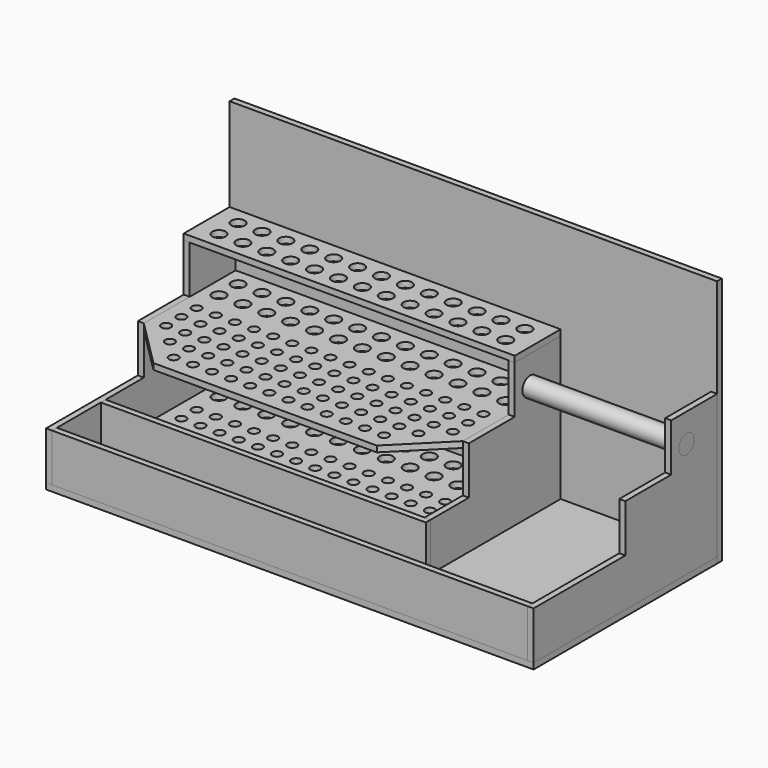
from build123d import *

# Parameters (mm, degrees)
F1_W           = 255
F1_H           = 120
F2_DEPTH       = 3.15
F4_DEPTH       = 3.15
F7_W           = 166.85
F7_H           = 3.15
F8_DEPTH       = 60
F8_DEPTH_BACK  = 25
F9_W           = 166.85
F9_H           = 3.15
F10_DEPTH      = 60
F10_DEPTH_BACK = 25
F11_W          = 255
F11_H          = 130
F12_DEPTH      = 3.15
F13_W          = 248.7
F13_H          = 25
F14_DEPTH      = 3.15
F15_W          = 35
F15_H          = 25
F16_DEPTH      = 25
F17_W          = 170
F17_H          = 25
F18_DEPTH      = 3.15
F20_DEPTH      = 25
F21_W          = 173.15
F21_H          = 30
F22_DEPTH      = 3.15
F23_R          = 3.5
F23_R_2        = 2.5
F24_DEPTH      = 81.301
F25_R          = 5
F26_DEPTH      = 255.001
F27_R          = 5
F28_DEPTH      = 85


with BuildPart() as f2:
    # F1 (on Top) → F2 (new body)
    with BuildSketch(Plane.XY):
        with Locations((127.5, 60)):
            Rectangle(F1_W, F1_H)
    extrude(amount=F2_DEPTH)


with BuildPart() as f4:
    # F3 (on face) → F4 (new body)
    with BuildSketch(Plane(origin=(0, 0, 0), x_dir=(0, -1, 0), z_dir=(-1, 0, 0))):
        Polygon((-120, 3.15), (0, 3.15), (0, 28.15), (-60, 28.15), (-60, 53.15), (-90, 53.15), (-90, 78.15), (-120, 78.15), align=None)
    extrude(amount=-F4_DEPTH)


with BuildPart() as f5_1:
    # F5: copy of F4
    add(f4.part.moved(Location((251.85, 0, 0))))


with BuildPart() as f6_1:
    # F6: copy of F4
    add(f4.part.moved(Location((170, 0, 0))))

    # F15 (on face) → F16 (cut)
    with BuildSketch(Plane.YZ.offset(173.15)):
        with Locations((17.5, 15.65)):
            Rectangle(F15_W, F15_H)
    extrude(amount=-F16_DEPTH, mode=Mode.SUBTRACT)


with BuildPart() as f8:
    # F7 (on face) → F8 (new body, two sides)
    with BuildSketch(Plane.XZ.offset(-60)) as f8_sk:
        with Locations((86.575, 4.725)):
            Rectangle(F7_W, F7_H)
    extrude(amount=-F8_DEPTH)
    extrude(f8_sk.sketch, amount=F8_DEPTH_BACK)


with BuildPart() as f10:
    # F9 (on face) → F10 (new body, two sides)
    with BuildSketch(Plane.XZ.offset(-60)) as f10_sk:
        with Locations((86.575, 51.575)):
            Rectangle(F9_W, F9_H)
    extrude(amount=-F10_DEPTH)
    extrude(f10_sk.sketch, amount=F10_DEPTH_BACK)

    # F19 (on face) → F20 (cut)
    with BuildSketch(Plane.XY.offset(53.15)):
        Polygon((28.15, 35), (3.15, 60), (3.15, 35), align=None)
        Polygon((170, 35), (170, 60), (145, 35), align=None)
    extrude(amount=-F20_DEPTH, mode=Mode.SUBTRACT)


with BuildPart() as f12:
    # F11 (on face) → F12 (new body)
    with BuildSketch(Plane(origin=(0, 120, 0), x_dir=(-1, 0, 0), z_dir=(0, 1, 0))):
        with Locations((-127.5, 65)):
            Rectangle(F11_W, F11_H)
    extrude(amount=F12_DEPTH)


with BuildPart() as f14:
    # F13 (on face) → F14 (new body)
    with BuildSketch(Plane.XZ):
        with Locations((127.5, 15.65)):
            Rectangle(F13_W, F13_H)
    extrude(amount=-F14_DEPTH)


with BuildPart() as f18:
    # F17 (on face) → F18 (new body)
    with BuildSketch(Plane.XZ.offset(-35)):
        with Locations((88.15, 15.65)):
            Rectangle(F17_W, F17_H)
    extrude(amount=F18_DEPTH)


with BuildPart() as f22:
    # F21 (on face) → F22 (new body)
    with BuildSketch(Plane.XY.offset(78.15)):
        with Locations((86.575, 105)):
            Rectangle(F21_W, F21_H)
    extrude(amount=F22_DEPTH)


with BuildPart() as f24_tool:
    # F23 (on face) → F24 (new body, through all)
    with BuildSketch(Plane.XY.offset(81.3)):
        with Locations((11.575, 111.0924071222)):
            Circle(F23_R)
        with Locations((11.575, 98.5924071222)):
            Circle(F23_R)
        with Locations((24.075, 111.0924071222)):
            Circle(F23_R)
        with Locations((24.075, 98.5924071222)):
            Circle(F23_R)
        with Locations((36.575, 111.0924071222)):
            Circle(F23_R)
        with Locations((36.575, 98.5924071222)):
            Circle(F23_R)
        with Locations((49.075, 111.0924071222)):
            Circle(F23_R)
        with Locations((49.075, 98.5924071222)):
            Circle(F23_R)
        with Locations((61.575, 111.0924071222)):
            Circle(F23_R)
        with Locations((61.575, 98.5924071222)):
            Circle(F23_R)
        with Locations((74.075, 111.0924071222)):
            Circle(F23_R)
        with Locations((74.075, 98.5924071222)):
            Circle(F23_R)
        with Locations((86.575, 111.0924071222)):
            Circle(F23_R)
        with Locations((86.575, 98.5924071222)):
            Circle(F23_R)
        with Locations((99.075, 111.0924071222)):
            Circle(F23_R)
        with Locations((99.075, 98.5924071222)):
            Circle(F23_R)
        with Locations((111.575, 111.0924071222)):
            Circle(F23_R)
        with Locations((111.575, 98.5924071222)):
            Circle(F23_R)
        with Locations((124.075, 111.0924071222)):
            Circle(F23_R)
        with Locations((124.075, 98.5924071222)):
            Circle(F23_R)
        with Locations((136.575, 111.0924071222)):
            Circle(F23_R)
        with Locations((136.575, 98.5924071222)):
            Circle(F23_R)
        with Locations((149.075, 111.0924071222)):
            Circle(F23_R)
        with Locations((149.075, 98.5924071222)):
            Circle(F23_R)
        with Locations((161.575, 111.0924071222)):
            Circle(F23_R)
        with Locations((161.575, 98.5924071222)):
            Circle(F23_R)
        with Locations((11.575, 84)):
            Circle(F23_R_2)
        with Locations((11.575, 74)):
            Circle(F23_R_2)
        with Locations((11.575, 64)):
            Circle(F23_R_2)
        with Locations((21.575, 84)):
            Circle(F23_R_2)
        with Locations((21.575, 74)):
            Circle(F23_R_2)
        with Locations((21.575, 64)):
            Circle(F23_R_2)
        with Locations((31.575, 84)):
            Circle(F23_R_2)
        with Locations((31.575, 74)):
            Circle(F23_R_2)
        with Locations((31.575, 64)):
            Circle(F23_R_2)
        with Locations((41.575, 84)):
            Circle(F23_R_2)
        with Locations((41.575, 74)):
            Circle(F23_R_2)
        with Locations((41.575, 64)):
            Circle(F23_R_2)
        with Locations((51.575, 84)):
            Circle(F23_R_2)
        with Locations((51.575, 74)):
            Circle(F23_R_2)
        with Locations((51.575, 64)):
            Circle(F23_R_2)
        with Locations((61.575, 84)):
            Circle(F23_R_2)
        with Locations((61.575, 74)):
            Circle(F23_R_2)
        with Locations((61.575, 64)):
            Circle(F23_R_2)
        with Locations((71.575, 84)):
            Circle(F23_R_2)
        with Locations((71.575, 74)):
            Circle(F23_R_2)
        with Locations((71.575, 64)):
            Circle(F23_R_2)
        with Locations((81.575, 84)):
            Circle(F23_R_2)
        with Locations((81.575, 74)):
            Circle(F23_R_2)
        with Locations((81.575, 64)):
            Circle(F23_R_2)
        with Locations((91.575, 84)):
            Circle(F23_R_2)
        with Locations((91.575, 74)):
            Circle(F23_R_2)
        with Locations((91.575, 64)):
            Circle(F23_R_2)
        with Locations((101.575, 84)):
            Circle(F23_R_2)
        with Locations((101.575, 74)):
            Circle(F23_R_2)
        with Locations((101.575, 64)):
            Circle(F23_R_2)
        with Locations((111.575, 84)):
            Circle(F23_R_2)
        with Locations((111.575, 74)):
            Circle(F23_R_2)
        with Locations((111.575, 64)):
            Circle(F23_R_2)
        with Locations((121.575, 84)):
            Circle(F23_R_2)
        with Locations((121.575, 74)):
            Circle(F23_R_2)
        with Locations((121.575, 64)):
            Circle(F23_R_2)
        with Locations((131.575, 84)):
            Circle(F23_R_2)
        with Locations((131.575, 74)):
            Circle(F23_R_2)
        with Locations((131.575, 64)):
            Circle(F23_R_2)
        with Locations((21.575, 54)):
            Circle(F23_R_2)
        with Locations((31.575, 54)):
            Circle(F23_R_2)
        with Locations((41.575, 54)):
            Circle(F23_R_2)
        with Locations((51.575, 54)):
            Circle(F23_R_2)
        with Locations((61.575, 54)):
            Circle(F23_R_2)
        with Locations((71.575, 54)):
            Circle(F23_R_2)
        with Locations((81.575, 54)):
            Circle(F23_R_2)
        with Locations((91.575, 54)):
            Circle(F23_R_2)
        with Locations((101.575, 54)):
            Circle(F23_R_2)
        with Locations((111.575, 54)):
            Circle(F23_R_2)
        with Locations((121.575, 54)):
            Circle(F23_R_2)
        with Locations((131.575, 54)):
            Circle(F23_R_2)
        with Locations((141.575, 84)):
            Circle(F23_R_2)
        with Locations((141.575, 74)):
            Circle(F23_R_2)
        with Locations((141.575, 64)):
            Circle(F23_R_2)
        with Locations((141.575, 54)):
            Circle(F23_R_2)
        with Locations((151.575, 84)):
            Circle(F23_R_2)
        with Locations((151.575, 74)):
            Circle(F23_R_2)
        with Locations((151.575, 64)):
            Circle(F23_R_2)
        with Locations((151.575, 54)):
            Circle(F23_R_2)
        with Locations((161.575, 84)):
            Circle(F23_R_2)
        with Locations((161.575, 74)):
            Circle(F23_R_2)
        with Locations((161.575, 64)):
            Circle(F23_R_2)
        with Locations((31.575, 44)):
            Circle(F23_R_2)
        with Locations((41.575, 44)):
            Circle(F23_R_2)
        with Locations((51.575, 44)):
            Circle(F23_R_2)
        with Locations((61.575, 44)):
            Circle(F23_R_2)
        with Locations((71.575, 44)):
            Circle(F23_R_2)
        with Locations((81.575, 44)):
            Circle(F23_R_2)
        with Locations((91.575, 44)):
            Circle(F23_R_2)
        with Locations((101.575, 44)):
            Circle(F23_R_2)
        with Locations((111.575, 44)):
            Circle(F23_R_2)
        with Locations((121.575, 44)):
            Circle(F23_R_2)
        with Locations((131.575, 44)):
            Circle(F23_R_2)
        with Locations((141.575, 44)):
            Circle(F23_R_2)
    extrude(amount=-F24_DEPTH)


with BuildPart() as f8_1:
    add(f8.part)

    # F24: cut by f24_tool
    add(f24_tool.part, mode=Mode.SUBTRACT)


with BuildPart() as f10_1:
    add(f10.part)

    # F24: cut by f24_tool
    add(f24_tool.part, mode=Mode.SUBTRACT)


with BuildPart() as f22_1:
    add(f22.part)

    # F24: cut by f24_tool
    add(f24_tool.part, mode=Mode.SUBTRACT)


with BuildPart() as f26_tool:
    # F25 (on face) → F26 (new body, through all)
    with BuildSketch(Plane.YZ.offset(255)):
        with Locations((100, 63.15)):
            Circle(F25_R)
    extrude(amount=-F26_DEPTH)


with BuildPart() as f5_1_1:
    add(f5_1.part)

    # F26: cut by f26_tool
    add(f26_tool.part, mode=Mode.SUBTRACT)


with BuildPart() as f6_1_1:
    add(f6_1.part)

    # F26: cut by f26_tool
    add(f26_tool.part, mode=Mode.SUBTRACT)


with BuildPart() as f28:
    # F27 (on face) → F28 (new body, through all)
    with BuildSketch(Plane.YZ.offset(255)):
        with Locations((100, 63.15)):
            Circle(F27_R)
    extrude(amount=-F28_DEPTH)


solid = Compound([f2.part, f4.part, f12.part, f14.part, f18.part, f8_1.part, f10_1.part, f22_1.part, f5_1_1.part, f6_1_1.part, f28.part])
